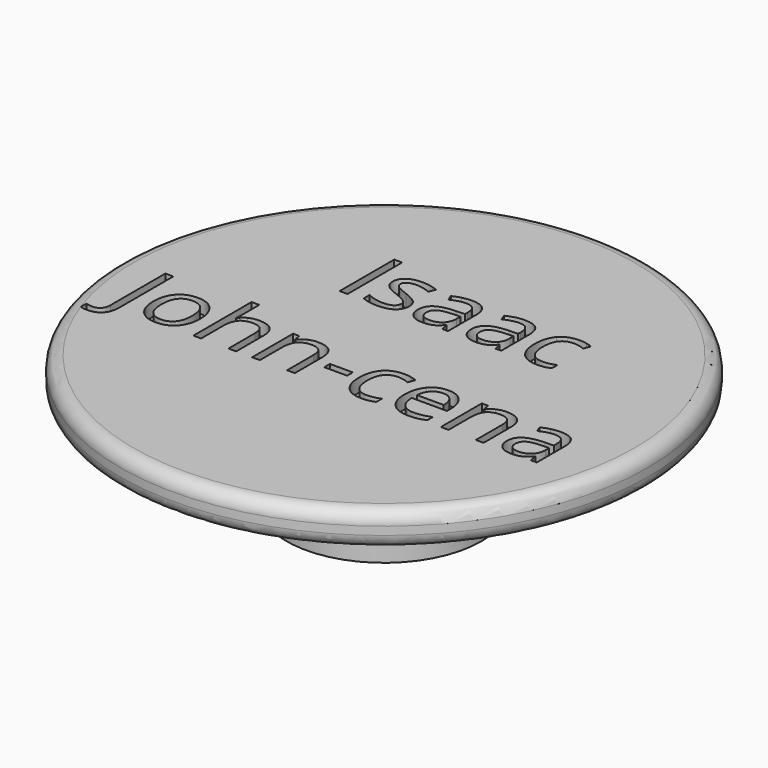
from build123d import *

# Parameters (mm, degrees)
F0_W     = 3.7
F0_H     = 3
F2_R     = 10
F2_W     = 0.868919099
F2_H     = 0.269059043
F2_W_2   = 0.3007796881
F2_H_2   = 2.5880647741
F3_DEPTH = 0.5
F4_R     = 0.5


with BuildPart() as f1:
    # F0 (on Front) → F1 (revolve)
    with BuildSketch(Plane.XZ):
        Polygon((10, 0), (0, 0), (0, -1.5), (3.7, -1.5), (10, -0.75), align=None)
        with Locations((1.85, -3)):
            Rectangle(F0_W, F0_H)
    revolve(axis=Axis((0, 0, -3), (0, 0, -1)))

    # F2 (on face) → F3 (join)
    with BuildSketch(Plane.XY):
        Circle(F2_R)
        with BuildLine():
            add(Edge.make_bspline(
                [(-8.1929409631, -3.0369352259), (-8.3628729903, -3.2218779155), (-8.6817787613, -3.2218779155)],
                knots=[0, 0, 0, 1, 1, 1], degree=2))
            add(Edge.make_bspline(
                [(-8.6817787613, -3.2218779155), (-8.8477457078, -3.2218779155), (-8.9434740832, -3.1742969479)],
                knots=[0, 0, 0, 1, 1, 1], degree=2))
            Line((-8.9434740832, -3.1742969479), (-8.9434740832, -2.9176995868))
            add(Edge.make_bspline(
                [(-8.9434740832, -2.9176995868), (-8.817724383, -2.9528188725), (-8.6817787613, -2.9528188725)],
                knots=[0, 0, 0, 1, 1, 1], degree=2))
            add(Edge.make_bspline(
                [(-8.6817787613, -2.9528188725), (-8.5061823332, -2.9528188725), (-8.4149854786, -2.8466113555)],
                knots=[0, 0, 0, 1, 1, 1], degree=2))
            add(Edge.make_bspline(
                [(-8.4149854786, -2.8466113555), (-8.323788624, -2.7404038385), (-8.323788624, -2.5404504865)],
                knots=[0, 0, 0, 1, 1, 1], degree=2))
            Line((-8.323788624, -2.5404504865), (-8.323788624, 0.0476142876))
            Line((-8.323788624, 0.0476142876), (-8.0230089359, 0.0476142876))
            Line((-8.0230089359, 0.0476142876), (-8.0230089359, -2.5155271225))
            add(Edge.make_bspline(
                [(-8.0230089359, -2.5155271225), (-8.0230089359, -2.8519925363), (-8.1929409631, -3.0369352259)],
                knots=[0, 0, 0, 1, 1, 1], degree=2))
        make_face(mode=Mode.SUBTRACT)
        with BuildLine():
            add(Edge.make_bspline(
                [(-5.9461563436, -0.8357490337), (-5.7062689652, -1.1067906171), (-5.7062689652, -1.568439291)],
                knots=[0, 0, 0, 1, 1, 1], degree=2))
            add(Edge.make_bspline(
                [(-5.7062689652, -1.568439291), (-5.7062689652, -2.0431160869), (-5.9450234634, -2.3096261495)],
                knots=[0, 0, 0, 1, 1, 1], degree=2))
            add(Edge.make_bspline(
                [(-5.9450234634, -2.3096261495), (-6.1837779616, -2.5761362122), (-6.605209389, -2.5761362122)],
                knots=[0, 0, 0, 1, 1, 1], degree=2))
            add(Edge.make_bspline(
                [(-6.605209389, -2.5761362122), (-6.8657718307, -2.5761362122), (-7.067424503, -2.4537851526)],
                knots=[0, 0, 0, 1, 1, 1], degree=2))
            add(Edge.make_bspline(
                [(-7.067424503, -2.4537851526), (-7.2690771753, -2.331434093), (-7.3789665528, -2.1031587365)],
                knots=[0, 0, 0, 1, 1, 1], degree=2))
            add(Edge.make_bspline(
                [(-7.3789665528, -2.1031587365), (-7.4888559304, -1.87488338), (-7.4888559304, -1.568439291)],
                knots=[0, 0, 0, 1, 1, 1], degree=2))
            add(Edge.make_bspline(
                [(-7.4888559304, -1.568439291), (-7.4888559304, -1.0943289351), (-7.2515175324, -0.8295181927)],
                knots=[0, 0, 0, 1, 1, 1], degree=2))
            add(Edge.make_bspline(
                [(-7.2515175324, -0.8295181927), (-7.0141791345, -0.5647074504), (-6.592747707, -0.5647074504)],
                knots=[0, 0, 0, 1, 1, 1], degree=2))
            add(Edge.make_bspline(
                [(-6.592747707, -0.5647074504), (-6.186043722, -0.5647074504), (-5.9461563436, -0.8357490337)],
                knots=[0, 0, 0, 1, 1, 1], degree=2))
        make_face(mode=Mode.SUBTRACT)
        with BuildLine():
            Line((-3.5690905033, -2.5404504865), (-3.8630729103, -2.5404504865))
            Line((-3.8630729103, -2.5404504865), (-3.8630729103, -1.2852192456))
            add(Edge.make_bspline(
                [(-3.8630729103, -1.2852192456), (-3.8630729103, -1.0484472878), (-3.9709797476, -0.931477409)],
                knots=[0, 0, 0, 1, 1, 1], degree=2))
            add(Edge.make_bspline(
                [(-3.9709797476, -0.931477409), (-4.0788865848, -0.8145075303), (-4.3094277017, -0.8145075303)],
                knots=[0, 0, 0, 1, 1, 1], degree=2))
            add(Edge.make_bspline(
                [(-4.3094277017, -0.8145075303), (-4.6153053507, -0.8145075303), (-4.7560657132, -0.981040917)],
                knots=[0, 0, 0, 1, 1, 1], degree=2))
            add(Edge.make_bspline(
                [(-4.7560657132, -0.981040917), (-4.8968260757, -1.1475743036), (-4.8968260757, -1.5259562842)],
                knots=[0, 0, 0, 1, 1, 1], degree=2))
            Line((-4.8968260757, -1.5259562842), (-4.8968260757, -2.5404504865))
            Line((-4.8968260757, -2.5404504865), (-5.1908084827, -2.5404504865))
            Line((-5.1908084827, -2.5404504865), (-5.1908084827, 0.2141476743))
            Line((-5.1908084827, 0.2141476743), (-4.8968260757, 0.2141476743))
            Line((-4.8968260757, 0.2141476743), (-4.8968260757, -0.6196521391))
            add(Edge.make_bspline(
                [(-4.8968260757, -0.6196521391), (-4.8968260757, -0.7703252033), (-4.910987078, -0.8694522191)],
                knots=[0, 0, 0, 1, 1, 1], degree=2))
            Line((-4.910987078, -0.8694522191), (-4.8934274352, -0.8694522191))
            add(Edge.make_bspline(
                [(-4.8934274352, -0.8694522191), (-4.8067621013, -0.7295415167), (-4.6464595556, -0.6491070239)],
                knots=[0, 0, 0, 1, 1, 1], degree=2))
            add(Edge.make_bspline(
                [(-4.6464595556, -0.6491070239), (-4.48615701, -0.568672531), (-4.2811056972, -0.568672531)],
                knots=[0, 0, 0, 1, 1, 1], degree=2))
            add(Edge.make_bspline(
                [(-4.2811056972, -0.568672531), (-3.9253813203, -0.568672531), (-3.7472359118, -0.737754898)],
                knots=[0, 0, 0, 1, 1, 1], degree=2))
            add(Edge.make_bspline(
                [(-3.7472359118, -0.737754898), (-3.5690905033, -0.9068372651), (-3.5690905033, -1.275023324)],
                knots=[0, 0, 0, 1, 1, 1], degree=2))
            Line((-3.5690905033, -1.275023324), (-3.5690905033, -2.5404504865))
        make_face(mode=Mode.SUBTRACT)
        with BuildLine():
            Line((-1.3441138273, -2.5404504865), (-1.6380962343, -2.5404504865))
            Line((-1.6380962343, -2.5404504865), (-1.6380962343, -1.2852192456))
            add(Edge.make_bspline(
                [(-1.6380962343, -1.2852192456), (-1.6380962343, -1.0484472878), (-1.7460030716, -0.931477409)],
                knots=[0, 0, 0, 1, 1, 1], degree=2))
            add(Edge.make_bspline(
                [(-1.7460030716, -0.931477409), (-1.8539099088, -0.8145075303), (-2.0844510257, -0.8145075303)],
                knots=[0, 0, 0, 1, 1, 1], degree=2))
            add(Edge.make_bspline(
                [(-2.0844510257, -0.8145075303), (-2.3886293544, -0.8145075303), (-2.530239377, -0.9790583766)],
                knots=[0, 0, 0, 1, 1, 1], degree=2))
            add(Edge.make_bspline(
                [(-2.530239377, -0.9790583766), (-2.6718493997, -1.143609223), (-2.6718493997, -1.5225576436)],
                knots=[0, 0, 0, 1, 1, 1], degree=2))
            Line((-2.6718493997, -1.5225576436), (-2.6718493997, -2.5404504865))
            Line((-2.6718493997, -2.5404504865), (-2.9658318067, -2.5404504865))
            Line((-2.9658318067, -2.5404504865), (-2.9658318067, -0.6003931761))
            Line((-2.9658318067, -0.6003931761), (-2.7267940885, -0.6003931761))
            Line((-2.7267940885, -0.6003931761), (-2.6792131209, -0.8660535786))
            Line((-2.6792131209, -0.8660535786), (-2.6650521186, -0.8660535786))
            add(Edge.make_bspline(
                [(-2.6650521186, -0.8660535786), (-2.5744217041, -0.7227442356), (-2.4115701781, -0.643725843)],
                knots=[0, 0, 0, 1, 1, 1], degree=2))
            add(Edge.make_bspline(
                [(-2.4115701781, -0.643725843), (-2.248718652, -0.5647074504), (-2.0487653, -0.5647074504)],
                knots=[0, 0, 0, 1, 1, 1], degree=2))
            add(Edge.make_bspline(
                [(-2.0487653, -0.5647074504), (-1.6981388839, -0.5647074504), (-1.5211263556, -0.7337898174)],
                knots=[0, 0, 0, 1, 1, 1], degree=2))
            add(Edge.make_bspline(
                [(-1.5211263556, -0.7337898174), (-1.3441138273, -0.9028721845), (-1.3441138273, -1.275023324)],
                knots=[0, 0, 0, 1, 1, 1], degree=2))
            Line((-1.3441138273, -1.275023324), (-1.3441138273, -2.5404504865))
        make_face(mode=Mode.SUBTRACT)
        with Locations((-0.4689638872, -1.568722511)):
            Rectangle(F2_W, F2_H, mode=Mode.SUBTRACT)
        with BuildLine():
            add(Edge.make_bspline(
                [(1.6908721783, -2.474743436), (1.4965832272, -2.5761362122), (1.2009014999, -2.5761362122)],
                knots=[0, 0, 0, 1, 1, 1], degree=2))
            add(Edge.make_bspline(
                [(1.2009014999, -2.5761362122), (0.7794700725, -2.5761362122), (0.5483625155, -2.3167066507)],
                knots=[0, 0, 0, 1, 1, 1], degree=2))
            add(Edge.make_bspline(
                [(0.5483625155, -2.3167066507), (0.3172549586, -2.0572770892), (0.3172549586, -1.5826002932)],
                knots=[0, 0, 0, 1, 1, 1], degree=2))
            add(Edge.make_bspline(
                [(0.3172549586, -1.5826002932), (0.3172549586, -1.0960282554), (0.5520443761, -0.8303678529)],
                knots=[0, 0, 0, 1, 1, 1], degree=2))
            add(Edge.make_bspline(
                [(0.5520443761, -0.8303678529), (0.7868337937, -0.5647074504), (1.220160463, -0.5647074504)],
                knots=[0, 0, 0, 1, 1, 1], degree=2))
            add(Edge.make_bspline(
                [(1.220160463, -0.5647074504), (1.3600711654, -0.5647074504), (1.4999818678, -0.5950119952)],
                knots=[0, 0, 0, 1, 1, 1], degree=2))
            add(Edge.make_bspline(
                [(1.4999818678, -0.5950119952), (1.6398925702, -0.6253165401), (1.7191941829, -0.6661002266)],
                knots=[0, 0, 0, 1, 1, 1], degree=2))
            Line((1.7191941829, -0.6661002266), (1.6291302085, -0.9153338665))
            add(Edge.make_bspline(
                [(1.6291302085, -0.9153338665), (1.5317025129, -0.8762495002), (1.4167151745, -0.8507596961)],
                knots=[0, 0, 0, 1, 1, 1], degree=2))
            add(Edge.make_bspline(
                [(1.4167151745, -0.8507596961), (1.3017278361, -0.825269892), (1.2133631819, -0.825269892)],
                knots=[0, 0, 0, 1, 1, 1], degree=2))
            add(Edge.make_bspline(
                [(1.2133631819, -0.825269892), (0.6219997273, -0.825269892), (0.6219997273, -1.5792016527)],
                knots=[0, 0, 0, 1, 1, 1], degree=2))
            add(Edge.make_bspline(
                [(0.6219997273, -1.5792016527), (0.6219997273, -1.9366253499), (0.7661587304, -2.1277988804)],
                knots=[0, 0, 0, 1, 1, 1], degree=2))
            add(Edge.make_bspline(
                [(0.7661587304, -2.1277988804), (0.9103177334, -2.318972411), (1.1935377788, -2.318972411)],
                knots=[0, 0, 0, 1, 1, 1], degree=2))
            add(Edge.make_bspline(
                [(1.1935377788, -2.318972411), (1.4359741376, -2.318972411), (1.6908721783, -2.2147474344)],
                knots=[0, 0, 0, 1, 1, 1], degree=2))
            Line((1.6908721783, -2.2147474344), (1.6908721783, -2.474743436))
        make_face(mode=Mode.SUBTRACT)
        with BuildLine():
            add(Edge.make_bspline(
                [(3.3063593168, -2.5466813275), (3.1675814946, -2.5761362122), (2.9710267832, -2.5761362122)],
                knots=[0, 0, 0, 1, 1, 1], degree=2))
            add(Edge.make_bspline(
                [(2.9710267832, -2.5761362122), (2.5410987544, -2.5761362122), (2.2921483345, -2.3138744502)],
                knots=[0, 0, 0, 1, 1, 1], degree=2))
            add(Edge.make_bspline(
                [(2.2921483345, -2.3138744502), (2.0431979147, -2.0516126883), (2.0431979147, -1.5865653739)],
                knots=[0, 0, 0, 1, 1, 1], degree=2))
            add(Edge.make_bspline(
                [(2.0431979147, -1.5865653739), (2.0431979147, -1.1169865387), (2.2743054717, -0.8408469945)],
                knots=[0, 0, 0, 1, 1, 1], degree=2))
            add(Edge.make_bspline(
                [(2.2743054717, -0.8408469945), (2.5054130287, -0.5647074504), (2.895123811, -0.5647074504)],
                knots=[0, 0, 0, 1, 1, 1], degree=2))
            add(Edge.make_bspline(
                [(2.895123811, -0.5647074504), (3.2593447893, -0.5647074504), (3.4717598233, -0.8045948287)],
                knots=[0, 0, 0, 1, 1, 1], degree=2))
            add(Edge.make_bspline(
                [(3.4717598233, -0.8045948287), (3.6841748573, -1.0444822071), (3.6841748573, -1.43759163)],
                knots=[0, 0, 0, 1, 1, 1], degree=2))
            Line((3.6841748573, -1.43759163), (3.6841748573, -1.6233839797))
            Line((3.6841748573, -1.6233839797), (2.3479426835, -1.6233839797))
            add(Edge.make_bspline(
                [(2.3479426835, -1.6233839797), (2.3570057249, -1.9649473544), (2.5207069111, -2.1419598827)],
                knots=[0, 0, 0, 1, 1, 1], degree=2))
            add(Edge.make_bspline(
                [(2.5207069111, -2.1419598827), (2.6844080973, -2.318972411), (2.9817891449, -2.318972411)],
                knots=[0, 0, 0, 1, 1, 1], degree=2))
            add(Edge.make_bspline(
                [(2.9817891449, -2.318972411), (3.295030515, -2.318972411), (3.6009081639, -2.1881247501)],
                knots=[0, 0, 0, 1, 1, 1], degree=2))
            Line((3.6009081639, -2.1881247501), (3.6009081639, -2.4503865121))
            add(Edge.make_bspline(
                [(3.6009081639, -2.4503865121), (3.445137139, -2.5172264428), (3.3063593168, -2.5466813275)],
                knots=[0, 0, 0, 1, 1, 1], degree=2))
        make_face(mode=Mode.SUBTRACT)
        with BuildLine():
            Line((5.8071923169, -2.5404504865), (5.5132099099, -2.5404504865))
            Line((5.5132099099, -2.5404504865), (5.5132099099, -1.2852192456))
            add(Edge.make_bspline(
                [(5.5132099099, -1.2852192456), (5.5132099099, -1.0484472878), (5.4053030726, -0.931477409)],
                knots=[0, 0, 0, 1, 1, 1], degree=2))
            add(Edge.make_bspline(
                [(5.4053030726, -0.931477409), (5.2973962354, -0.8145075303), (5.0668551185, -0.8145075303)],
                knots=[0, 0, 0, 1, 1, 1], degree=2))
            add(Edge.make_bspline(
                [(5.0668551185, -0.8145075303), (4.7626767898, -0.8145075303), (4.6210667672, -0.9790583766)],
                knots=[0, 0, 0, 1, 1, 1], degree=2))
            add(Edge.make_bspline(
                [(4.6210667672, -0.9790583766), (4.4794567445, -1.143609223), (4.4794567445, -1.5225576436)],
                knots=[0, 0, 0, 1, 1, 1], degree=2))
            Line((4.4794567445, -1.5225576436), (4.4794567445, -2.5404504865))
            Line((4.4794567445, -2.5404504865), (4.1854743375, -2.5404504865))
            Line((4.1854743375, -2.5404504865), (4.1854743375, -0.6003931761))
            Line((4.1854743375, -0.6003931761), (4.4245120557, -0.6003931761))
            Line((4.4245120557, -0.6003931761), (4.4720930233, -0.8660535786))
            Line((4.4720930233, -0.8660535786), (4.4862540256, -0.8660535786))
            add(Edge.make_bspline(
                [(4.4862540256, -0.8660535786), (4.5768844401, -0.7227442356), (4.7397359662, -0.643725843)],
                knots=[0, 0, 0, 1, 1, 1], degree=2))
            add(Edge.make_bspline(
                [(4.7397359662, -0.643725843), (4.9025874922, -0.5647074504), (5.1025408442, -0.5647074504)],
                knots=[0, 0, 0, 1, 1, 1], degree=2))
            add(Edge.make_bspline(
                [(5.1025408442, -0.5647074504), (5.4531672603, -0.5647074504), (5.6301797886, -0.7337898174)],
                knots=[0, 0, 0, 1, 1, 1], degree=2))
            add(Edge.make_bspline(
                [(5.6301797886, -0.7337898174), (5.8071923169, -0.9028721845), (5.8071923169, -1.275023324)],
                knots=[0, 0, 0, 1, 1, 1], degree=2))
            Line((5.8071923169, -1.275023324), (5.8071923169, -2.5404504865))
        make_face(mode=Mode.SUBTRACT)
        with BuildLine():
            Line((7.8214532792, -2.5404504865), (7.6033738443, -2.5404504865))
            Line((7.6033738443, -2.5404504865), (7.545030515, -2.2640277222))
            Line((7.545030515, -2.2640277222), (7.5308695127, -2.2640277222))
            add(Edge.make_bspline(
                [(7.5308695127, -2.2640277222), (7.3858608495, -2.4464214314), (7.2417018465, -2.5112788218)],
                knots=[0, 0, 0, 1, 1, 1], degree=2))
            add(Edge.make_bspline(
                [(7.2417018465, -2.5112788218), (7.0975428434, -2.5761362122), (6.8811627288, -2.5761362122)],
                knots=[0, 0, 0, 1, 1, 1], degree=2))
            add(Edge.make_bspline(
                [(6.8811627288, -2.5761362122), (6.5928447227, -2.5761362122), (6.4291435365, -2.4271624683)],
                knots=[0, 0, 0, 1, 1, 1], degree=2))
            add(Edge.make_bspline(
                [(6.4291435365, -2.4271624683), (6.2654423503, -2.2781887245), (6.2654423503, -2.0040317206)],
                knots=[0, 0, 0, 1, 1, 1], degree=2))
            add(Edge.make_bspline(
                [(6.2654423503, -2.0040317206), (6.2654423503, -1.4166333467), (7.2051664606, -1.3883113421)],
                knots=[0, 0, 0, 1, 1, 1], degree=2))
            Line((7.2051664606, -1.3883113421), (7.5342681533, -1.3775489804))
            Line((7.5342681533, -1.3775489804), (7.5342681533, -1.2568972411))
            add(Edge.make_bspline(
                [(7.5342681533, -1.2568972411), (7.5342681533, -1.0286218846), (7.4362740176, -0.9198653872)],
                knots=[0, 0, 0, 1, 1, 1], degree=2))
            add(Edge.make_bspline(
                [(7.4362740176, -0.9198653872), (7.3382798819, -0.8111088898), (7.1218997673, -0.8111088898)],
                knots=[0, 0, 0, 1, 1, 1], degree=2))
            add(Edge.make_bspline(
                [(7.1218997673, -0.8111088898), (6.8794634085, -0.8111088898), (6.5735857596, -0.9595161935)],
                knots=[0, 0, 0, 1, 1, 1], degree=2))
            Line((6.5735857596, -0.9595161935), (6.4829553451, -0.7346394775))
            add(Edge.make_bspline(
                [(6.4829553451, -0.7346394775), (6.626264688, -0.6570371851), (6.7970463753, -0.6128548581)],
                knots=[0, 0, 0, 1, 1, 1], degree=2))
            add(Edge.make_bspline(
                [(6.7970463753, -0.6128548581), (6.9678280626, -0.568672531), (7.1400258502, -0.568672531)],
                knots=[0, 0, 0, 1, 1, 1], degree=2))
            add(Edge.make_bspline(
                [(7.1400258502, -0.568672531), (7.4866871857, -0.568672531), (7.6540702324, -0.7224610156)],
                knots=[0, 0, 0, 1, 1, 1], degree=2))
            add(Edge.make_bspline(
                [(7.6540702324, -0.7224610156), (7.8214532792, -0.8762495002), (7.8214532792, -1.2161135546)],
                knots=[0, 0, 0, 1, 1, 1], degree=2))
            Line((7.8214532792, -1.2161135546), (7.8214532792, -2.5404504865))
        make_face(mode=Mode.SUBTRACT)
        with Locations((-3.4441904633, 3.6838764494)):
            Rectangle(F2_W_2, F2_H_2, mode=Mode.SUBTRACT)
        with BuildLine():
            add(Edge.make_bspline(
                [(-1.4981855319, 3.2395041983), (-1.3769673525, 3.1120551779), (-1.3769673525, 2.918899107)],
                knots=[0, 0, 0, 1, 1, 1], degree=2))
            add(Edge.make_bspline(
                [(-1.3769673525, 2.918899107), (-1.3769673525, 2.6481407437), (-1.5786200248, 2.5011495402)],
                knots=[0, 0, 0, 1, 1, 1], degree=2))
            add(Edge.make_bspline(
                [(-1.5786200248, 2.5011495402), (-1.780272697, 2.3541583367), (-2.1450601154, 2.3541583367)],
                knots=[0, 0, 0, 1, 1, 1], degree=2))
            add(Edge.make_bspline(
                [(-2.1450601154, 2.3541583367), (-2.5308058171, 2.3541583367), (-2.7466194917, 2.4765093962)],
                knots=[0, 0, 0, 1, 1, 1], degree=2))
            Line((-2.7466194917, 2.4765093962), (-2.7466194917, 2.7489670798))
            add(Edge.make_bspline(
                [(-2.7466194917, 2.7489670798), (-2.6067087893, 2.6781620685), (-2.4466894637, 2.637661602)],
                knots=[0, 0, 0, 1, 1, 1], degree=2))
            add(Edge.make_bspline(
                [(-2.4466894637, 2.637661602), (-2.2866701381, 2.5971611355), (-2.1376963942, 2.5971611355)],
                knots=[0, 0, 0, 1, 1, 1], degree=2))
            add(Edge.make_bspline(
                [(-2.1376963942, 2.5971611355), (-1.9077217174, 2.5971611355), (-1.7839545576, 2.6705151273)],
                knots=[0, 0, 0, 1, 1, 1], degree=2))
            add(Edge.make_bspline(
                [(-1.7839545576, 2.6705151273), (-1.6601873978, 2.743869119), (-1.6601873978, 2.8945421831)],
                knots=[0, 0, 0, 1, 1, 1], degree=2))
            add(Edge.make_bspline(
                [(-1.6601873978, 2.8945421831), (-1.6601873978, 3.0078302013), (-1.7581815335, 3.0882646941)],
                knots=[0, 0, 0, 1, 1, 1], degree=2))
            add(Edge.make_bspline(
                [(-1.7581815335, 3.0882646941), (-1.8561756692, 3.168699187), (-2.1416614749, 3.2785885646)],
                knots=[0, 0, 0, 1, 1, 1], degree=2))
            add(Edge.make_bspline(
                [(-2.1416614749, 3.2785885646), (-2.4124198382, 3.3794149007), (-2.5265575165, 3.4547514328)],
                knots=[0, 0, 0, 1, 1, 1], degree=2))
            add(Edge.make_bspline(
                [(-2.5265575165, 3.4547514328), (-2.6406951947, 3.5300879648), (-2.6964895436, 3.6255331201)],
                knots=[0, 0, 0, 1, 1, 1], degree=2))
            add(Edge.make_bspline(
                [(-2.6964895436, 3.6255331201), (-2.7522838926, 3.7209782754), (-2.7522838926, 3.8535252566)],
                knots=[0, 0, 0, 1, 1, 1], degree=2))
            add(Edge.make_bspline(
                [(-2.7522838926, 3.8535252566), (-2.7522838926, 4.0908636545), (-2.5591278217, 4.2282253765)],
                knots=[0, 0, 0, 1, 1, 1], degree=2))
            add(Edge.make_bspline(
                [(-2.5591278217, 4.2282253765), (-2.3659717508, 4.3655870985), (-2.030072777, 4.3655870985)],
                knots=[0, 0, 0, 1, 1, 1], degree=2))
            add(Edge.make_bspline(
                [(-2.030072777, 4.3655870985), (-1.7168314069, 4.3655870985), (-1.417184599, 4.2381380781)],
                knots=[0, 0, 0, 1, 1, 1], degree=2))
            Line((-1.417184599, 4.2381380781), (-1.5219760157, 3.9991003599))
            add(Edge.make_bspline(
                [(-1.5219760157, 3.9991003599), (-1.8136926624, 4.1191856591), (-2.0510310604, 4.1191856591)],
                knots=[0, 0, 0, 1, 1, 1], degree=2))
            add(Edge.make_bspline(
                [(-2.0510310604, 4.1191856591), (-2.2600474538, 4.1191856591), (-2.3662549708, 4.0537618286)],
                knots=[0, 0, 0, 1, 1, 1], degree=2))
            add(Edge.make_bspline(
                [(-2.3662549708, 4.0537618286), (-2.4724624878, 3.9883379981), (-2.4724624878, 3.8733506597)],
                knots=[0, 0, 0, 1, 1, 1], degree=2))
            add(Edge.make_bspline(
                [(-2.4724624878, 3.8733506597), (-2.4724624878, 3.7951819272), (-2.4325284614, 3.7405204585)],
                knots=[0, 0, 0, 1, 1, 1], degree=2))
            add(Edge.make_bspline(
                [(-2.4325284614, 3.7405204585), (-2.392594435, 3.6858589897), (-2.3042297809, 3.6362954818)],
                knots=[0, 0, 0, 1, 1, 1], degree=2))
            add(Edge.make_bspline(
                [(-2.3042297809, 3.6362954818), (-2.2158651267, 3.5867319739), (-1.9643657265, 3.4927029188)],
                knots=[0, 0, 0, 1, 1, 1], degree=2))
            add(Edge.make_bspline(
                [(-1.9643657265, 3.4927029188), (-1.6194037113, 3.3669532187), (-1.4981855319, 3.2395041983)],
                knots=[0, 0, 0, 1, 1, 1], degree=2))
        make_face(mode=Mode.SUBTRACT)
        with BuildLine():
            Line((0.5121103497, 2.3898440624), (0.2940309148, 2.3898440624))
            Line((0.2940309148, 2.3898440624), (0.2356875855, 2.6662668266))
            Line((0.2356875855, 2.6662668266), (0.2215265832, 2.6662668266))
            add(Edge.make_bspline(
                [(0.2215265832, 2.6662668266), (0.07651792, 2.4838731174), (-0.067641083, 2.419015727)],
                knots=[0, 0, 0, 1, 1, 1], degree=2))
            add(Edge.make_bspline(
                [(-0.067641083, 2.419015727), (-0.2118000861, 2.3541583367), (-0.4281802007, 2.3541583367)],
                knots=[0, 0, 0, 1, 1, 1], degree=2))
            add(Edge.make_bspline(
                [(-0.4281802007, 2.3541583367), (-0.7164982068, 2.3541583367), (-0.880199393, 2.5031320805)],
                knots=[0, 0, 0, 1, 1, 1], degree=2))
            add(Edge.make_bspline(
                [(-0.880199393, 2.5031320805), (-1.0439005792, 2.6521058243), (-1.0439005792, 2.9262628282)],
                knots=[0, 0, 0, 1, 1, 1], degree=2))
            add(Edge.make_bspline(
                [(-1.0439005792, 2.9262628282), (-1.0439005792, 3.5136612022), (-0.1041764689, 3.5419832067)],
                knots=[0, 0, 0, 1, 1, 1], degree=2))
            Line((-0.1041764689, 3.5419832067), (0.2249252238, 3.5527455684))
            Line((0.2249252238, 3.5527455684), (0.2249252238, 3.6733973077))
            add(Edge.make_bspline(
                [(0.2249252238, 3.6733973077), (0.2249252238, 3.9016726643), (0.1269310881, 4.0104291617)],
                knots=[0, 0, 0, 1, 1, 1], degree=2))
            add(Edge.make_bspline(
                [(0.1269310881, 4.0104291617), (0.0289369524, 4.1191856591), (-0.1874431622, 4.1191856591)],
                knots=[0, 0, 0, 1, 1, 1], degree=2))
            add(Edge.make_bspline(
                [(-0.1874431622, 4.1191856591), (-0.429879521, 4.1191856591), (-0.7357571699, 3.9707783553)],
                knots=[0, 0, 0, 1, 1, 1], degree=2))
            Line((-0.7357571699, 3.9707783553), (-0.8263875844, 4.1956550713))
            add(Edge.make_bspline(
                [(-0.8263875844, 4.1956550713), (-0.6830782415, 4.2732573637), (-0.5122965542, 4.3174396908)],
                knots=[0, 0, 0, 1, 1, 1], degree=2))
            add(Edge.make_bspline(
                [(-0.5122965542, 4.3174396908), (-0.3415148668, 4.3616220179), (-0.1693170793, 4.3616220179)],
                knots=[0, 0, 0, 1, 1, 1], degree=2))
            add(Edge.make_bspline(
                [(-0.1693170793, 4.3616220179), (0.1773442562, 4.3616220179), (0.344727303, 4.2078335333)],
                knots=[0, 0, 0, 1, 1, 1], degree=2))
            add(Edge.make_bspline(
                [(0.344727303, 4.2078335333), (0.5121103497, 4.0540450486), (0.5121103497, 3.7141809943)],
                knots=[0, 0, 0, 1, 1, 1], degree=2))
            Line((0.5121103497, 3.7141809943), (0.5121103497, 2.3898440624))
        make_face(mode=Mode.SUBTRACT)
        with BuildLine():
            Line((2.5280706323, 2.3898440624), (2.3099911974, 2.3898440624))
            Line((2.3099911974, 2.3898440624), (2.2516478681, 2.6662668266))
            Line((2.2516478681, 2.6662668266), (2.2374868658, 2.6662668266))
            add(Edge.make_bspline(
                [(2.2374868658, 2.6662668266), (2.0924782026, 2.4838731174), (1.9483191995, 2.419015727)],
                knots=[0, 0, 0, 1, 1, 1], degree=2))
            add(Edge.make_bspline(
                [(1.9483191995, 2.419015727), (1.8041601965, 2.3541583367), (1.5877800818, 2.3541583367)],
                knots=[0, 0, 0, 1, 1, 1], degree=2))
            add(Edge.make_bspline(
                [(1.5877800818, 2.3541583367), (1.2994620757, 2.3541583367), (1.1357608895, 2.5031320805)],
                knots=[0, 0, 0, 1, 1, 1], degree=2))
            add(Edge.make_bspline(
                [(1.1357608895, 2.5031320805), (0.9720597033, 2.6521058243), (0.9720597033, 2.9262628282)],
                knots=[0, 0, 0, 1, 1, 1], degree=2))
            add(Edge.make_bspline(
                [(0.9720597033, 2.9262628282), (0.9720597033, 3.5136612022), (1.9117838137, 3.5419832067)],
                knots=[0, 0, 0, 1, 1, 1], degree=2))
            Line((1.9117838137, 3.5419832067), (2.2408855063, 3.5527455684))
            Line((2.2408855063, 3.5527455684), (2.2408855063, 3.6733973077))
            add(Edge.make_bspline(
                [(2.2408855063, 3.6733973077), (2.2408855063, 3.9016726643), (2.1428913707, 4.0104291617)],
                knots=[0, 0, 0, 1, 1, 1], degree=2))
            add(Edge.make_bspline(
                [(2.1428913707, 4.0104291617), (2.044897235, 4.1191856591), (1.8285171204, 4.1191856591)],
                knots=[0, 0, 0, 1, 1, 1], degree=2))
            add(Edge.make_bspline(
                [(1.8285171204, 4.1191856591), (1.5860807616, 4.1191856591), (1.2802031126, 3.9707783553)],
                knots=[0, 0, 0, 1, 1, 1], degree=2))
            Line((1.2802031126, 3.9707783553), (1.1895726981, 4.1956550713))
            add(Edge.make_bspline(
                [(1.1895726981, 4.1956550713), (1.3328820411, 4.2732573637), (1.5036637284, 4.3174396908)],
                knots=[0, 0, 0, 1, 1, 1], degree=2))
            add(Edge.make_bspline(
                [(1.5036637284, 4.3174396908), (1.6744454157, 4.3616220179), (1.8466432033, 4.3616220179)],
                knots=[0, 0, 0, 1, 1, 1], degree=2))
            add(Edge.make_bspline(
                [(1.8466432033, 4.3616220179), (2.1933045387, 4.3616220179), (2.3606875855, 4.2078335333)],
                knots=[0, 0, 0, 1, 1, 1], degree=2))
            add(Edge.make_bspline(
                [(2.3606875855, 4.2078335333), (2.5280706323, 4.0540450486), (2.5280706323, 3.7141809943)],
                knots=[0, 0, 0, 1, 1, 1], degree=2))
            Line((2.5280706323, 3.7141809943), (2.5280706323, 2.3898440624))
        make_face(mode=Mode.SUBTRACT)
        with BuildLine():
            add(Edge.make_bspline(
                [(4.3984558115, 2.4555511129), (4.2041668605, 2.3541583367), (3.9084851332, 2.3541583367)],
                knots=[0, 0, 0, 1, 1, 1], degree=2))
            add(Edge.make_bspline(
                [(3.9084851332, 2.3541583367), (3.4870537057, 2.3541583367), (3.2559461487, 2.6135878982)],
                knots=[0, 0, 0, 1, 1, 1], degree=2))
            add(Edge.make_bspline(
                [(3.2559461487, 2.6135878982), (3.0248385918, 2.8730174597), (3.0248385918, 3.3476942556)],
                knots=[0, 0, 0, 1, 1, 1], degree=2))
            add(Edge.make_bspline(
                [(3.0248385918, 3.3476942556), (3.0248385918, 3.8342662935), (3.2596280093, 4.099926696)],
                knots=[0, 0, 0, 1, 1, 1], degree=2))
            add(Edge.make_bspline(
                [(3.2596280093, 4.099926696), (3.4944174269, 4.3655870985), (3.9277440962, 4.3655870985)],
                knots=[0, 0, 0, 1, 1, 1], degree=2))
            add(Edge.make_bspline(
                [(3.9277440962, 4.3655870985), (4.0676547986, 4.3655870985), (4.207565501, 4.3352825536)],
                knots=[0, 0, 0, 1, 1, 1], degree=2))
            add(Edge.make_bspline(
                [(4.207565501, 4.3352825536), (4.3474762034, 4.3049780088), (4.4267778161, 4.2641943223)],
                knots=[0, 0, 0, 1, 1, 1], degree=2))
            Line((4.4267778161, 4.2641943223), (4.3367138417, 4.0149606824))
            add(Edge.make_bspline(
                [(4.3367138417, 4.0149606824), (4.2392861461, 4.0540450486), (4.1242988077, 4.0795348527)],
                knots=[0, 0, 0, 1, 1, 1], degree=2))
            add(Edge.make_bspline(
                [(4.1242988077, 4.0795348527), (4.0093114693, 4.1050246568), (3.9209468151, 4.1050246568)],
                knots=[0, 0, 0, 1, 1, 1], degree=2))
            add(Edge.make_bspline(
                [(3.9209468151, 4.1050246568), (3.3295833605, 4.1050246568), (3.3295833605, 3.3510928962)],
                knots=[0, 0, 0, 1, 1, 1], degree=2))
            add(Edge.make_bspline(
                [(3.3295833605, 3.3510928962), (3.3295833605, 2.993669199), (3.4737423636, 2.8024956684)],
                knots=[0, 0, 0, 1, 1, 1], degree=2))
            add(Edge.make_bspline(
                [(3.4737423636, 2.8024956684), (3.6179013667, 2.6113221378), (3.901121412, 2.6113221378)],
                knots=[0, 0, 0, 1, 1, 1], degree=2))
            add(Edge.make_bspline(
                [(3.901121412, 2.6113221378), (4.1435577708, 2.6113221378), (4.3984558115, 2.7155471145)],
                knots=[0, 0, 0, 1, 1, 1], degree=2))
            Line((4.3984558115, 2.7155471145), (4.3984558115, 2.4555511129))
        make_face(mode=Mode.SUBTRACT)
        with BuildLine():
            add(Edge.make_bspline(
                [(-0.6394623545, 2.6801446088), (-0.5431675391, 2.5971611355), (-0.3698368714, 2.5971611355)],
                knots=[0, 0, 0, 1, 1, 1], degree=2))
            add(Edge.make_bspline(
                [(-0.3698368714, 2.5971611355), (-0.0951134274, 2.5971611355), (0.0615072576, 2.7475509796)],
                knots=[0, 0, 0, 1, 1, 1], degree=2))
            add(Edge.make_bspline(
                [(0.0615072576, 2.7475509796), (0.2181279427, 2.8979408237), (0.2181279427, 3.168699187)],
                knots=[0, 0, 0, 1, 1, 1], degree=2))
            Line((0.2181279427, 3.168699187), (0.2181279427, 3.343729175))
            Line((0.2181279427, 3.343729175), (-0.0758544643, 3.3318339331))
            add(Edge.make_bspline(
                [(-0.0758544643, 3.3318339331), (-0.4264808804, 3.3193722511), (-0.5811190252, 3.2227942156)],
                knots=[0, 0, 0, 1, 1, 1], degree=2))
            add(Edge.make_bspline(
                [(-0.5811190252, 3.2227942156), (-0.7357571699, 3.1262161802), (-0.7357571699, 2.9228641877)],
                knots=[0, 0, 0, 1, 1, 1], degree=2))
            add(Edge.make_bspline(
                [(-0.7357571699, 2.9228641877), (-0.7357571699, 2.7631280821), (-0.6394623545, 2.6801446088)],
                knots=[0, 0, 0, 1, 1, 1], degree=2))
        make_face()
        with BuildLine():
            add(Edge.make_bspline(
                [(1.376497928, 2.6801446088), (1.4727927434, 2.5971611355), (1.6461234112, 2.5971611355)],
                knots=[0, 0, 0, 1, 1, 1], degree=2))
            add(Edge.make_bspline(
                [(1.6461234112, 2.5971611355), (1.9208468551, 2.5971611355), (2.0774675402, 2.7475509796)],
                knots=[0, 0, 0, 1, 1, 1], degree=2))
            add(Edge.make_bspline(
                [(2.0774675402, 2.7475509796), (2.2340882253, 2.8979408237), (2.2340882253, 3.168699187)],
                knots=[0, 0, 0, 1, 1, 1], degree=2))
            Line((2.2340882253, 3.168699187), (2.2340882253, 3.343729175))
            Line((2.2340882253, 3.343729175), (1.9401058182, 3.3318339331))
            add(Edge.make_bspline(
                [(1.9401058182, 3.3318339331), (1.5894794021, 3.3193722511), (1.4348412574, 3.2227942156)],
                knots=[0, 0, 0, 1, 1, 1], degree=2))
            add(Edge.make_bspline(
                [(1.4348412574, 3.2227942156), (1.2802031126, 3.1262161802), (1.2802031126, 2.9228641877)],
                knots=[0, 0, 0, 1, 1, 1], degree=2))
            add(Edge.make_bspline(
                [(1.2802031126, 2.9228641877), (1.2802031126, 2.7631280821), (1.376497928, 2.6801446088)],
                knots=[0, 0, 0, 1, 1, 1], degree=2))
        make_face()
        with BuildLine():
            add(Edge.make_bspline(
                [(-7.0371199581, -1.0039817406), (-7.1841111617, -1.193455951), (-7.1841111617, -1.568439291)],
                knots=[0, 0, 0, 1, 1, 1], degree=2))
            add(Edge.make_bspline(
                [(-7.1841111617, -1.568439291), (-7.1841111617, -1.9405904305), (-7.0354206379, -2.1351626016)],
                knots=[0, 0, 0, 1, 1, 1], degree=2))
            add(Edge.make_bspline(
                [(-7.0354206379, -2.1351626016), (-6.8867301141, -2.3297347728), (-6.5984121079, -2.3297347728)],
                knots=[0, 0, 0, 1, 1, 1], degree=2))
            add(Edge.make_bspline(
                [(-6.5984121079, -2.3297347728), (-6.3095276617, -2.3297347728), (-6.1599874778, -2.1360122618)],
                knots=[0, 0, 0, 1, 1, 1], degree=2))
            add(Edge.make_bspline(
                [(-6.1599874778, -2.1360122618), (-6.0104472939, -1.9422897508), (-6.0104472939, -1.568439291)],
                knots=[0, 0, 0, 1, 1, 1], degree=2))
            add(Edge.make_bspline(
                [(-6.0104472939, -1.568439291), (-6.0104472939, -1.1985539118), (-6.1599874778, -1.006530721)],
                knots=[0, 0, 0, 1, 1, 1], degree=2))
            add(Edge.make_bspline(
                [(-6.1599874778, -1.006530721), (-6.3095276617, -0.8145075303), (-6.6018107485, -0.8145075303)],
                knots=[0, 0, 0, 1, 1, 1], degree=2))
            add(Edge.make_bspline(
                [(-6.6018107485, -0.8145075303), (-6.8901287546, -0.8145075303), (-7.0371199581, -1.0039817406)],
                knots=[0, 0, 0, 1, 1, 1], degree=2))
        make_face()
        with BuildLine():
            add(Edge.make_bspline(
                [(3.2454670071, -0.9589497534), (3.1216998473, -0.8111088898), (2.8911587304, -0.8111088898)],
                knots=[0, 0, 0, 1, 1, 1], degree=2))
            add(Edge.make_bspline(
                [(2.8911587304, -0.8111088898), (2.657785413, -0.8111088898), (2.5187243708, -0.9631980541)],
                knots=[0, 0, 0, 1, 1, 1], degree=2))
            add(Edge.make_bspline(
                [(2.5187243708, -0.9631980541), (2.3796633285, -1.1152872184), (2.3547399646, -1.3843462615)],
                knots=[0, 0, 0, 1, 1, 1], degree=2))
            Line((2.3547399646, -1.3843462615), (3.3692341669, -1.3843462615))
            add(Edge.make_bspline(
                [(3.3692341669, -1.3843462615), (3.3692341669, -1.1067906171), (3.2454670071, -0.9589497534)],
                knots=[0, 0, 0, 1, 1, 1], degree=2))
        make_face()
        with BuildLine():
            add(Edge.make_bspline(
                [(6.669880575, -2.25014994), (6.7661753904, -2.3331334133), (6.9395060581, -2.3331334133)],
                knots=[0, 0, 0, 1, 1, 1], degree=2))
            add(Edge.make_bspline(
                [(6.9395060581, -2.3331334133), (7.2142295021, -2.3331334133), (7.3708501871, -2.1827435692)],
                knots=[0, 0, 0, 1, 1, 1], degree=2))
            add(Edge.make_bspline(
                [(7.3708501871, -2.1827435692), (7.5274708722, -2.0323537252), (7.5274708722, -1.7615953619)],
                knots=[0, 0, 0, 1, 1, 1], degree=2))
            Line((7.5274708722, -1.7615953619), (7.5274708722, -1.5865653739))
            Line((7.5274708722, -1.5865653739), (7.2334884652, -1.5984606158))
            add(Edge.make_bspline(
                [(7.2334884652, -1.5984606158), (6.8828620491, -1.6109222977), (6.7282239043, -1.7075003332)],
                knots=[0, 0, 0, 1, 1, 1], degree=2))
            add(Edge.make_bspline(
                [(6.7282239043, -1.7075003332), (6.5735857596, -1.8040783687), (6.5735857596, -2.0074303612)],
                knots=[0, 0, 0, 1, 1, 1], degree=2))
            add(Edge.make_bspline(
                [(6.5735857596, -2.0074303612), (6.5735857596, -2.1671664667), (6.669880575, -2.25014994)],
                knots=[0, 0, 0, 1, 1, 1], degree=2))
        make_face()
    extrude(amount=F3_DEPTH)

    # F4
    f4_edges = [f1.edges().sort_by_distance(p)[0] for p in [
        (-10, 0, -0.75),
        (-10, 0, 0.5),
        (10, 0, -0.125),
    ]]
    fillet(f4_edges, radius=F4_R)


solid = f1.part
